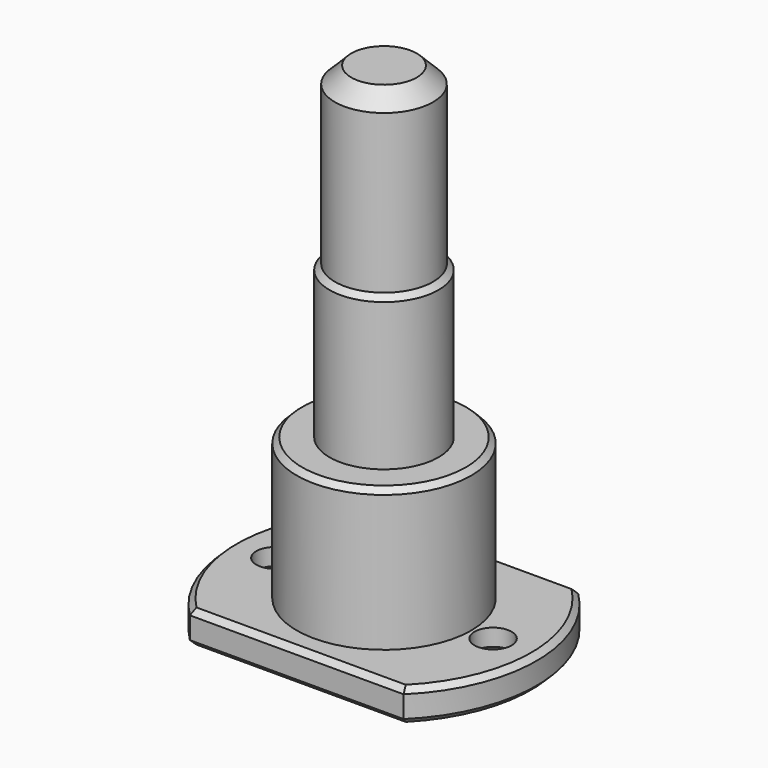
from build123d import *

# Parameters (mm, degrees)
F1_DEPTH       = 3
F2_D           = 3.4
F2_CSINK_D     = 6.3
F2_CSINK_ANGLE = 90
F3_R           = 8
F4_DEPTH       = 13
F5_R           = 5
F6_DEPTH       = 14
F7_R           = 4.5
F8_DEPTH       = 16
F9_SIZE        = 1.5
F10_SIZE       = 0.49999


# Not quite as in the source:
# - a fillet or chamfer is up to 0.001 mm smaller than in the source, because OpenCascade refuses the exact size


with BuildPart() as f1:
    # F0 (on Top) → F1 (new body)
    with BuildSketch(Plane.XY):
        with BuildLine():
            Line((9.7979589711, 10), (-9.7979589711, 10))
            ThreePointArc((-9.7979589711, 10), (-14, 0), (-9.7979589711, -10))
            Line((-9.7979589711, -10), (9.7979589711, -10))
            ThreePointArc((9.7979589711, -10), (14, 0), (9.7979589711, 10))
        make_face()
    extrude(amount=F1_DEPTH)

    # F2 (through all)
    with Locations(Plane(origin=(0, 0, 0), x_dir=(1, 0, 0), z_dir=(0, 0, -1))):
        with Locations((-10, 0), (10, 0)):
            CounterSinkHole(F2_D / 2, F2_CSINK_D / 2, counter_sink_angle=F2_CSINK_ANGLE)

    # F3 (on face) → F4 (join)
    with BuildSketch(Plane.XY.offset(3)):
        Circle(F3_R)
    extrude(amount=F4_DEPTH)

    # F5 (on face) → F6 (join)
    with BuildSketch(Plane.XY.offset(16)):
        Circle(F5_R)
    extrude(amount=F6_DEPTH)

    # F7 (on face) → F8 (join)
    with BuildSketch(Plane.XY.offset(30)):
        Circle(F7_R)
    extrude(amount=F8_DEPTH)

    # F9
    f9_edges = [f1.edges().sort_by_distance(p)[0] for p in [
        (-4.5, 0, 46),
    ]]
    chamfer(f9_edges, length=F9_SIZE)

    # F10 (size 0.5 in the source; OpenCascade refuses exactly that, so slightly less here)
    f10_edges = [f1.edges().sort_by_distance(p)[0] for p in [
        (-5, 0, 30),
        (0, -10, 3),
        (14, 0, 3),
        (0, 10, 3),
        (-14, 0, 3),
        (-14, 0, 0),
        (0, -10, 0),
        (14, 0, 0),
        (0, 10, 0),
        (-8, 0, 16),
    ]]
    chamfer(f10_edges, length=F10_SIZE)


solid = f1.part
